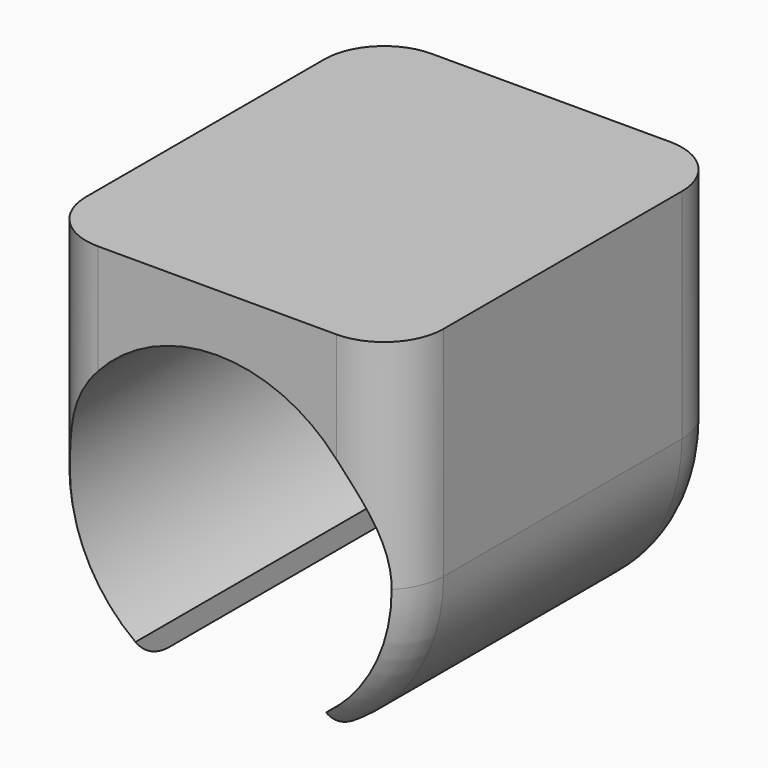
from build123d import *

# Parameters (mm, degrees)
F1_DEPTH     = 35
F2_T1_DEPTH  = 30.7885359973
F2_T4_ANGLE  = 105.523431357
F2_T6_ANGLE  = 105.523431357
F2_T8_ANGLE  = 105.523431357
F2_T10_ANGLE = 105.523431357


# Not quite as in the source:
# - a fillet or chamfer that OpenCascade refuses, or shapes differently, is made with other operations: its cross-section is extruded or revolved along the edge and cut away or added


with BuildPart() as f1:
    # F0 (on Front) → F1 (new body)
    with BuildSketch(Plane.XZ):
        with BuildLine():
            ThreePointArc((-8, -10.8742815855), (0, 13.5), (8, -10.8742815855))
            Line((8, -10.8742815855), (8, -12.6885775404))
            ThreePointArc((8, -12.6885775404), (13.1339255366, -7.2456883731), (15, 0))
            Line((15, 0), (15, 18.2885359973))
            Line((15, 18.2885359973), (-15, 18.2885359973))
            Line((-15, 18.2885359973), (-15, 0))
            ThreePointArc((-15, 0), (-13.1339255366, -7.2456883731), (-8, -12.6885775404))
            Line((-8, -12.6885775404), (-8, -10.8742815855))
        make_face()
    extrude(amount=F1_DEPTH)

    # F2: fillet of radius 5 on 4 edges, made by hand

    # F2_s2 → F2_t1 (cut)
    with BuildSketch(Plane.XY):
        with BuildLine():
            ThreePointArc((15, -30), (13.5355339059, -33.5355339059), (10, -35))
            Line((10, -35), (15, -35))
            Line((15, -35), (15, -30))
        make_face()
        with BuildLine():
            ThreePointArc((-15, -30), (-13.5355339059, -33.5355339059), (-10, -35))
            Line((-10, -35), (-15, -35))
            Line((-15, -35), (-15, -30))
        make_face()
        with BuildLine():
            ThreePointArc((15, -5), (13.5355339059, -1.4644660941), (10, 0))
            Line((10, 0), (15, 0))
            Line((15, 0), (15, -5))
        make_face()
        with BuildLine():
            ThreePointArc((-15, -5), (-13.5355339059, -1.4644660941), (-10, 0))
            Line((-10, 0), (-15, 0))
            Line((-15, 0), (-15, -5))
        make_face()
    extrude(amount=F2_T1_DEPTH, mode=Mode.SUBTRACT)

    # F2_s3 → F2_t4 (revolve, cut)
    with BuildSketch(Plane.XY):
        with BuildLine():
            ThreePointArc((-15, -5), (-13.5355339059, -1.4644660941), (-10, 0))
            Line((-10, 0), (-15, 0))
            Line((-15, 0), (-15, -5))
        make_face()
    revolve(axis=Axis((0, 0, 0), (0, -1, 0)), revolution_arc=F2_T4_ANGLE, mode=Mode.SUBTRACT)

    # F2_s5 → F2_t6 (revolve, cut)
    with BuildSketch(Plane(origin=(0, 0, 0), x_dir=(0, 1, 0), z_dir=(-0.9635210843, 0, 0.2676324346))):
        with BuildLine():
            ThreePointArc((-5, 15), (-1.4644660941, 13.5355339059), (0, 10))
            Line((0, 10), (0, 15))
            Line((0, 15), (-5, 15))
        make_face()
    revolve(axis=Axis((0, 0, 0), (0, -1, 0)), revolution_arc=F2_T6_ANGLE, mode=Mode.SUBTRACT)

    # F2_s7 → F2_t8 (revolve, cut)
    with BuildSketch(Plane.XY):
        with BuildLine():
            ThreePointArc((-15, -30), (-13.5355339059, -33.5355339059), (-10, -35))
            Line((-10, -35), (-15, -35))
            Line((-15, -35), (-15, -30))
        make_face()
    revolve(axis=Axis((0, -35, 0), (0, -1, 0)), revolution_arc=F2_T8_ANGLE, mode=Mode.SUBTRACT)

    # F2_s9 → F2_t10 (revolve, cut)
    with BuildSketch(Plane(origin=(0, 0, 0), x_dir=(0, 1, 0), z_dir=(-0.9635210843, 0, 0.2676324346))):
        with BuildLine():
            ThreePointArc((-30, 15), (-33.5355339059, 13.5355339059), (-35, 10))
            Line((-35, 10), (-35, 15))
            Line((-35, 15), (-30, 15))
        make_face()
    revolve(axis=Axis((0, -35, 0), (0, -1, 0)), revolution_arc=F2_T10_ANGLE, mode=Mode.SUBTRACT)


solid = f1.part
